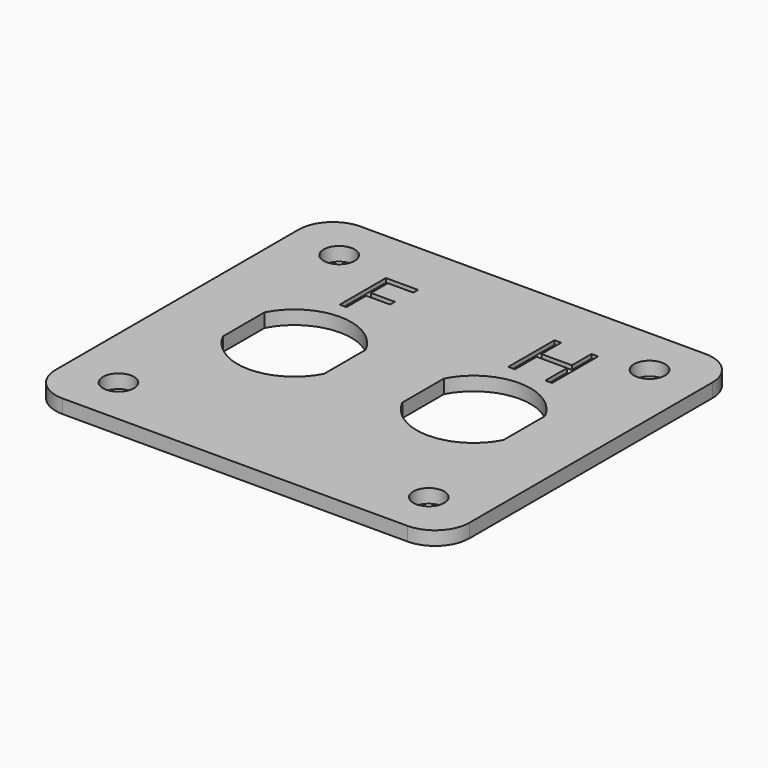
from build123d import *

# Parameters (mm, degrees)
F0_W         = 60
F0_H         = 54
F0_W_2       = 45
F0_H_2       = 40
F1_DEPTH     = 2
F2_D         = 4.5
F3_R         = 5
F4_TEXT_SIZE = 11.7097749353
F5_DEPTH     = 0.6


# Not quite as in the source:
# - a feature names something its author has since deleted; it is built from what else it names
# - Text() gives the source's letters only with a copy of the font that has no kerning and outlines rounded to 1/6400 em; it was checked with that copy


with BuildPart() as f1:
    # F0 (on Top) → F1 (new body)
    with BuildSketch(Plane.XY):
        Rectangle(F0_W, F0_H)
        Rectangle(F0_W_2, F0_H_2, mode=Mode.SUBTRACT)
        Rectangle(F0_W_2, F0_H_2)
        with BuildLine():
            ThreePointArc((-5.6602534446, 3.7670440005), (-4.9807915265, 1.9377294597), (-4.75, 0))
            ThreePointArc((-4.75, 0), (-4.9807915265, -1.9377294597), (-5.6602534446, -3.7670440005))
            ThreePointArc((-5.6602534446, -3.7670440005), (-13, -8.25), (-20.3397465554, -3.7670440005))
            ThreePointArc((-20.3397465554, -3.7670440005), (-21.25, 0), (-20.3397465554, 3.7670440005))
            ThreePointArc((-20.3397465554, 3.7670440005), (-13, 8.25), (-5.6602534446, 3.7670440005))
        make_face(mode=Mode.SUBTRACT)
        with BuildLine():
            ThreePointArc((20.3397465554, 3.7670440005), (21.0192084735, 1.9377294597), (21.25, 0))
            ThreePointArc((21.25, 0), (21.0192084735, -1.9377294597), (20.3397465554, -3.7670440005))
            ThreePointArc((20.3397465554, -3.7670440005), (13, -8.25), (5.6602534446, -3.7670440005))
            ThreePointArc((5.6602534446, -3.7670440005), (4.75, 0), (5.6602534446, 3.7670440005))
            ThreePointArc((5.6602534446, 3.7670440005), (13, 8.25), (20.3397465554, 3.7670440005))
        make_face(mode=Mode.SUBTRACT)
        with BuildLine():
            Line((-20.3397465554, -3.7670440005), (-20.3397465554, 3.7670440005))
            ThreePointArc((-20.3397465554, 3.7670440005), (-21.25, 0), (-20.3397465554, -3.7670440005))
        make_face()
        with BuildLine():
            ThreePointArc((-5.6602534446, -3.7670440005), (-4.9807915265, -1.9377294597), (-4.75, 0))
            ThreePointArc((-4.75, 0), (-4.9807915265, 1.9377294597), (-5.6602534446, 3.7670440005))
            Line((-5.6602534446, 3.7670440005), (-5.6602534446, -3.7670440005))
        make_face()
        with BuildLine():
            Line((5.6602534446, -3.7670440005), (5.6602534446, 3.7670440005))
            ThreePointArc((5.6602534446, 3.7670440005), (4.75, 0), (5.6602534446, -3.7670440005))
        make_face()
        with BuildLine():
            ThreePointArc((20.3397465554, -3.7670440005), (21.0192084735, -1.9377294597), (21.25, 0))
            ThreePointArc((21.25, 0), (21.0192084735, 1.9377294597), (20.3397465554, 3.7670440005))
            Line((20.3397465554, 3.7670440005), (20.3397465554, -3.7670440005))
        make_face()
    extrude(amount=F1_DEPTH)

    # F2 (through all)
    with Locations(Plane(origin=(0, 0, 0), x_dir=(1, 0, 0), z_dir=(0, 0, -1))):
        with Locations((-22.5, -20), (-22.5, 20), (22.5, 20), (22.5, -20)):
            Hole(F2_D / 2)

    # F3
    f3_edges = [f1.edges().sort_by_distance(p)[0] for p in [
        (-30, -27, 1),
        (30, -27, 1),
        (30, 27, 1),
        (-30, 27, 1),
    ]]
    fillet(f3_edges, radius=F3_R)

    # F4 (on face) → F5 (cut)
    with BuildSketch(Plane.XY.offset(2)):
        with Locations((-16.0185516616, 10.5711127908)):
            Text('F', F4_TEXT_SIZE, font='Open Sans', text_align=(TextAlign.LEFT, TextAlign.BOTTOM))
        with Locations((8.4101939574, 10.5711127908)):
            Text('H', F4_TEXT_SIZE, font='Open Sans', text_align=(TextAlign.LEFT, TextAlign.BOTTOM))
    extrude(amount=-F5_DEPTH, mode=Mode.SUBTRACT)


solid = f1.part
